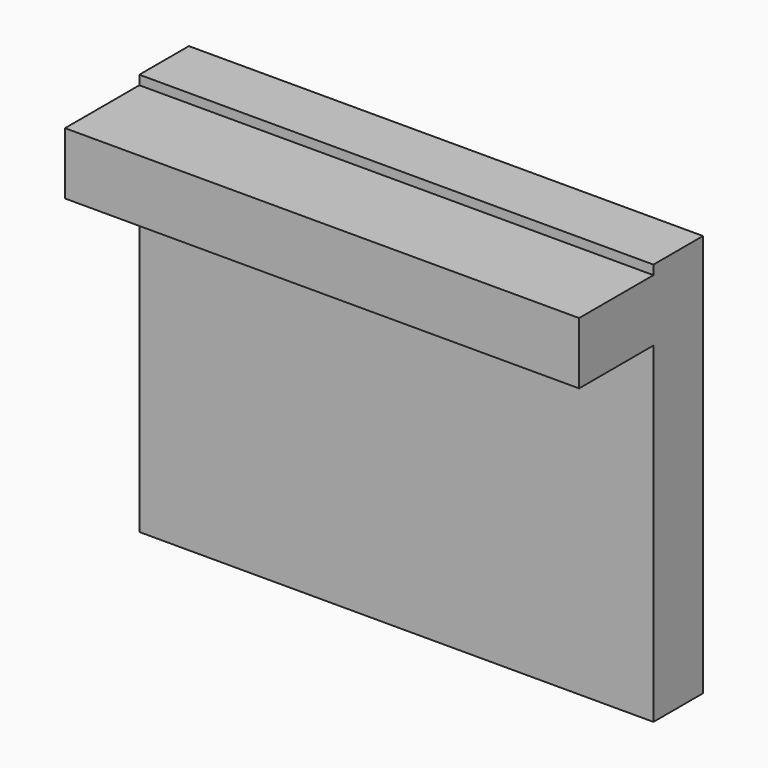
from build123d import *

# Parameters (mm, degrees)
F0_W     = 83
F0_H     = 10
F1_DEPTH = 65
F2_W     = 83
F2_H     = 10
F3_DEPTH = 15


# Not quite as in the source:
# - a feature names something its author has since deleted; it is built from what else it names


with BuildPart() as f1:
    # F0 (on Top) → F1 (new body)
    with BuildSketch(Plane.XY):
        Rectangle(F0_W, F0_H)
    extrude(amount=F1_DEPTH)

    # F2 (on face) → F3 (join)
    with BuildSketch(Plane.XZ.offset(5)):
        with Locations((0, 58.5)):
            Rectangle(F2_W, F2_H)
    extrude(amount=F3_DEPTH)


solid = f1.part
